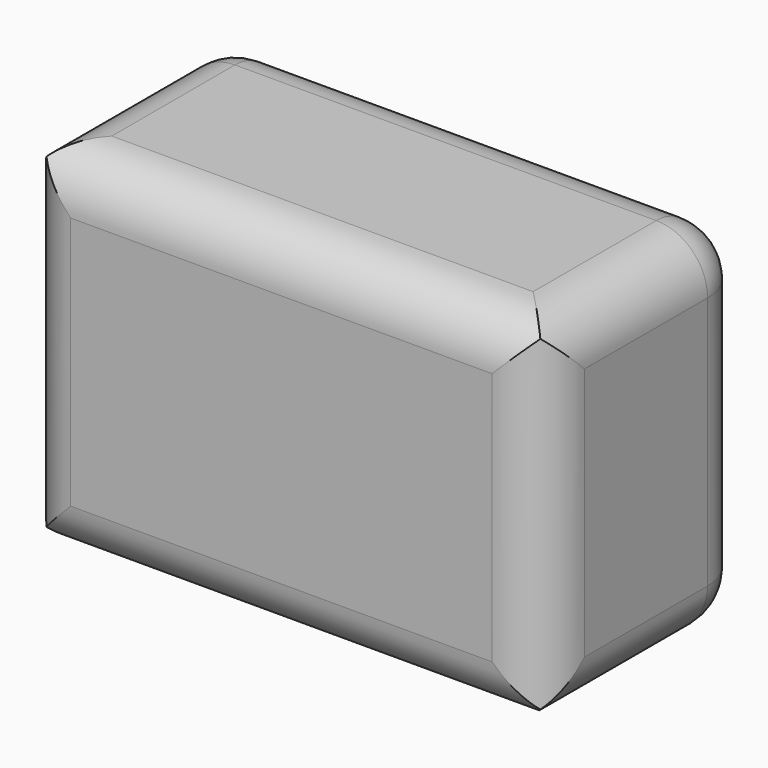
from build123d import *

# Parameters (mm, degrees)
F0_W         = 51.0475635529
F0_H         = 34.7123146057
F1_DEPTH     = 25
F2_R         = 5
F3_T1_DEPTH  = 50
F3_T3_DEPTH  = 76.0475635529
F4_T1_DEPTH  = 41.0475635528
F4_T3_DEPTH  = 24.7123146058
F4_S7_W      = 5
F4_S7_H      = 5
F4_T8_DEPTH  = 5
F4_S13_W     = 5
F4_S13_H     = 5
F4_T14_DEPTH = 5
F4_T18_ANGLE = 90.0000000014
F4_T20_ANGLE = 90.0000000014
F5_T1_DEPTH  = 49.7123146058


# Not quite as in the source:
# - a fillet or chamfer that OpenCascade refuses, or shapes differently, is made with other operations: its cross-section is extruded or revolved along the edge and cut away or added


with BuildPart() as f1:
    # F0 (on Front) → F1 (new body)
    with BuildSketch(Plane.XZ):
        Rectangle(F0_W, F0_H)
    extrude(amount=F1_DEPTH)

    # F2
    f2_edges = [f1.edges().sort_by_distance(p)[0] for p in [
        (0, -25, 17.356157),
        (0, 0, 17.356157),
        (-25.523782, -12.5, 17.356157),
        (25.523782, -12.5, 17.356157),
    ]]
    fillet(f2_edges, radius=F2_R)

    # F3: fillet of radius 5 on 4 edges, made by hand

    # F3_s2 → F3_t1 (cut)
    with BuildSketch(Plane.XZ.offset(-12.5)):
        with BuildLine():
            ThreePointArc((-25.5237817764, -12.3561573029), (-24.0593156824, -15.8916912088), (-20.5237817764, -17.3561573029))
            Line((-20.5237817764, -17.3561573029), (-25.5237817764, -17.3561573029))
            Line((-25.5237817764, -17.3561573029), (-25.5237817764, -12.3561573029))
        make_face()
        with BuildLine():
            ThreePointArc((25.5237817764, -12.3561573029), (24.0593156824, -15.8916912088), (20.5237817764, -17.3561573029))
            Line((20.5237817764, -17.3561573029), (25.5237817764, -17.3561573029))
            Line((25.5237817764, -17.3561573029), (25.5237817764, -12.3561573029))
        make_face()
    extrude(amount=F3_T1_DEPTH, mode=Mode.SUBTRACT)

    # F3_s4 → F3_t3 (cut)
    with BuildSketch(Plane.YZ.offset(-38.0237817764)):
        with BuildLine():
            ThreePointArc((-25, -12.3561573029), (-23.5355339059, -15.8916912088), (-20, -17.3561573029))
            Line((-20, -17.3561573029), (-25, -17.3561573029))
            Line((-25, -17.3561573029), (-25, -12.3561573029))
        make_face()
    extrude(amount=F3_T3_DEPTH, mode=Mode.SUBTRACT)

    # F4: fillet of radius 5 on 3 edges, made by hand

    # F4_s2 → F4_t1 (cut)
    with BuildSketch(Plane.YZ.offset(-20.5237817764)):
        with BuildLine():
            ThreePointArc((0, -12.3561573029), (-1.4644660941, -15.8916912088), (-5, -17.3561573029))
            Line((-5, -17.3561573029), (0, -17.3561573029))
            Line((0, -17.3561573029), (0, -12.3561573029))
        make_face()
    extrude(amount=F4_T1_DEPTH, mode=Mode.SUBTRACT)

    # F4_s4 → F4_t3 (cut)
    with BuildSketch(Plane.XY.offset(-12.3561573029)):
        with BuildLine():
            ThreePointArc((25.5237817764, -5), (24.0593156824, -1.4644660941), (20.5237817764, 0))
            Line((20.5237817764, 0), (25.5237817764, 0))
            Line((25.5237817764, 0), (25.5237817764, -5))
        make_face()
        with BuildLine():
            ThreePointArc((-25.5237817764, -5), (-24.0593156824, -1.4644660941), (-20.5237817764, 0))
            Line((-20.5237817764, 0), (-25.5237817764, 0))
            Line((-25.5237817764, 0), (-25.5237817764, -5))
        make_face()
    extrude(amount=F4_T3_DEPTH, mode=Mode.SUBTRACT)


with BuildPart() as f4_tool6:
    # F4_s7 → F4_t8 (new body)
    with BuildSketch(Plane.YZ.offset(20.5237817764)):
        with Locations((-2.5, 14.8561573029)):
            Rectangle(F4_S7_W, F4_S7_H)
    extrude(amount=F4_T8_DEPTH)

    # F4_s9 → F4_t10 (revolve, cut)
    with BuildSketch(Plane(origin=(20.5237817764, -5, 12.3561573029), x_dir=(0, -0.7071067812, -0.7071067812), z_dir=(0, -0.7071067812, 0.7071067812))):
        with BuildLine():
            ThreePointArc((0, -5), (5, 0), (0, 5))
            Line((0, 5), (0, -5))
        make_face()
    revolve(axis=Axis((20.5237817764, -5, 12.3561573029), (1, 0, 0)), mode=Mode.SUBTRACT)


with BuildPart() as f1_1:
    add(f1.part)

    # F4_t5: cut F4_tool6
    add(f4_tool6.part, mode=Mode.SUBTRACT)


with BuildPart() as f4_tool12:
    # F4_s13 → F4_t14 (new body)
    with BuildSketch(Plane.YZ.offset(-20.5237817764)):
        with Locations((-2.5, 14.8561573029)):
            Rectangle(F4_S13_W, F4_S13_H)
    extrude(amount=-F4_T14_DEPTH)

    # F4_s15 → F4_t16 (revolve, cut)
    with BuildSketch(Plane(origin=(-20.5237817764, -5, 12.3561573029), x_dir=(0, -0.7071067812, -0.7071067812), z_dir=(0, 0.7071067812, -0.7071067812))):
        with BuildLine():
            ThreePointArc((0, -5), (5, 0), (0, 5))
            Line((0, 5), (0, -5))
        make_face()
    revolve(axis=Axis((-20.5237817764, -5, 12.3561573029), (-1, 0, 0)), mode=Mode.SUBTRACT)


with BuildPart() as f1_2:
    add(f1_1.part)

    # F4_t11: cut F4_tool12
    add(f4_tool12.part, mode=Mode.SUBTRACT)

    # F4_s17 → F4_t18 (revolve, cut)
    with BuildSketch(Plane.YZ.offset(-20.5237817765)):
        with BuildLine():
            ThreePointArc((0, -12.3561573029), (-1.4644660941, -15.8916912088), (-5, -17.3561573029))
            Line((-5, -17.3561573029), (0, -17.3561573029))
            Line((0, -17.3561573029), (0, -12.3561573029))
        make_face()
    revolve(axis=Axis((-20.5237817765, 0, -12.356157303), (0, 1, 0)), revolution_arc=F4_T18_ANGLE, mode=Mode.SUBTRACT)

    # F4_s19 → F4_t20 (revolve, cut)
    with BuildSketch(Plane.XY.offset(-12.356157303)):
        with BuildLine():
            ThreePointArc((20.5237817764, 0), (24.0593156823, -1.4644660941), (25.5237817764, -5))
            Line((25.5237817764, -5), (25.5237817764, 0))
            Line((25.5237817764, 0), (20.5237817764, 0))
        make_face()
    revolve(axis=Axis((20.5237817765, 0, -12.356157303), (0, 1, 0)), revolution_arc=F4_T20_ANGLE, mode=Mode.SUBTRACT)

    # F5: fillet of radius 5 on 4 edges, made by hand

    # F5_s2 → F5_t1 (cut)
    with BuildSketch(Plane.XY.offset(-24.8561573029)):
        with BuildLine():
            ThreePointArc((20.5237817764, -25), (24.0593156824, -23.5355339059), (25.5237817764, -20))
            Line((25.5237817764, -20), (25.5237817764, -25))
            Line((25.5237817764, -25), (20.5237817764, -25))
        make_face()
        with BuildLine():
            ThreePointArc((-20.5237817764, -25), (-24.0593156824, -23.5355339059), (-25.5237817764, -20))
            Line((-25.5237817764, -20), (-25.5237817764, -25))
            Line((-25.5237817764, -25), (-20.5237817764, -25))
        make_face()
    extrude(amount=F5_T1_DEPTH, mode=Mode.SUBTRACT)


solid = f1_2.part
